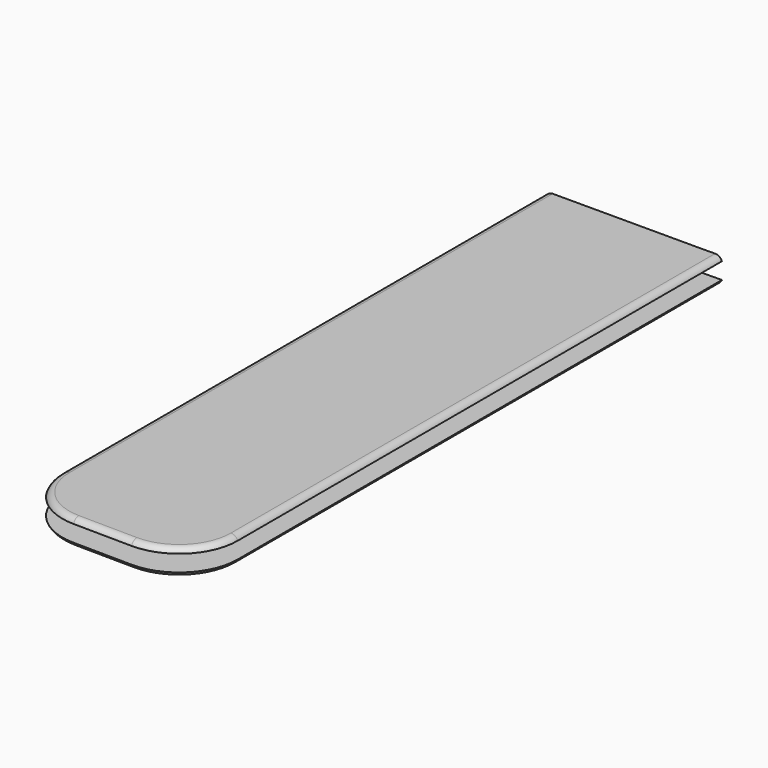
from build123d import *

# Parameters (mm, degrees)
F1_DEPTH        = 3.5
F2_DEPTH        = 2.25
F3_T1_DEPTH     = 169.9016407579
F3_T3_DEPTH     = 16.0006816658
F3_T5_DEPTH     = 169.6351240544
F3_T8_ANGLE     = 90.7094753215
F3_T10_ANGLE    = 89.290335423
F3_S1_T1_DEPTH  = 169.9016407579
F3_S1_T3_DEPTH  = 16.0006816658
F3_S1_T5_DEPTH  = 169.6351240544
F3_S1_T8_ANGLE  = 90.7094753215
F3_S1_T10_ANGLE = 89.290335423


# Not quite as in the source:
# - a fillet or chamfer that OpenCascade refuses, or shapes differently, is made with other operations: its cross-section is extruded or revolved along the edge and cut away or added


with BuildPart() as f1:
    # F0 (on Top) → F1 (new body, symmetric)
    with BuildSketch(Plane.XY):
        with BuildLine():
            Line((18, 42.4503772799), (-18, 42.4503772799))
            Line((-18, 42.4503772799), (-24.0000008941, 42.4503772799))
            Line((-24.0000008941, 42.4503772799), (-24.0000008941, -122.5496227201))
            ThreePointArc((-24.0000008941, -122.5496227201), (-19.3835574329, -133.7930496347), (-8.1981706793, -138.5483963291))
            Line((-8.1981706793, -138.5483963291), (7.8012836493, -138.7465754402))
            ThreePointArc((7.8012836493, -138.7465754402), (19.2428624423, -134.1313778333), (23.9994552225, -122.7478546813))
            Line((23.9994552225, -122.7478546813), (24.0000011197, 42.5186620212))
            Line((24.0000011197, 42.5186620212), (18, 42.4503772799))
        make_face()
    extrude(amount=F1_DEPTH, both=True)

    # F0 (on Top) → F2 (cut, symmetric)
    with BuildSketch(Plane.XY):
        with BuildLine():
            Line((18, 42.4503772799), (-18, 42.4503772799))
            Line((-18, 42.4503772799), (-24.0000008941, 42.4503772799))
            Line((-24.0000008941, 42.4503772799), (-24.0000008941, -122.5496227201))
            ThreePointArc((-24.0000008941, -122.5496227201), (-19.3835574329, -133.7930496347), (-8.1981706793, -138.5483963291))
            Line((-8.1981706793, -138.5483963291), (7.8012836493, -138.7465754402))
            ThreePointArc((7.8012836493, -138.7465754402), (19.2428624423, -134.1313778333), (23.9994552225, -122.7478546813))
            Line((23.9994552225, -122.7478546813), (24.0000011197, 42.5186620212))
            Line((24.0000011197, 42.5186620212), (18, 42.4503772799))
        make_face()
    extrude(amount=F2_DEPTH, both=True, mode=Mode.SUBTRACT)

    # F3: fillet of radius 2 on 1 edges, made by hand

    # F3_s2 → F3_t1 (cut)
    with BuildSketch(Plane(origin=(-0.0004054521, -122.7477754066, 0), x_dir=(0, 0, 1), z_dir=(3.3031e-06, 1, 0))):
        with BuildLine():
            ThreePointArc((-2.25, 23.9998606748), (-3.1583123952, 23.2638450417), (-3.5, 22.145811053))
            Line((-3.5, 22.145811053), (-3.5, 23.9998606748))
            Line((-3.5, 23.9998606748), (-2.25, 23.9998606748))
        make_face()
    extrude(amount=F3_T1_DEPTH, mode=Mode.SUBTRACT)

    # F3_s4 → F3_t3 (cut)
    with BuildSketch(Plane(origin=(-6.4810304011, 0.0802780406, 0), x_dir=(0, 0, 1), z_dir=(0.9999232947, -0.0123856668, 0))):
        with BuildLine():
            ThreePointArc((-3.5, 136.7852591194), (-3.1583123952, 137.9032931082), (-2.25, 138.6393087412))
            Line((-2.25, 138.6393087412), (-3.5, 138.6393087412))
            Line((-3.5, 138.6393087412), (-3.5, 136.7852591194))
        make_face()
    extrude(amount=F3_T3_DEPTH, mode=Mode.SUBTRACT)

    # F3_s6 → F3_t5 (cut)
    with BuildSketch(Plane.XZ.offset(-47.0855013343)):
        with BuildLine():
            ThreePointArc((-22.1459512723, -3.5), (-23.263985261, -3.1583123952), (-24.0000008941, -2.25))
            Line((-24.0000008941, -2.25), (-24.0000008941, -3.5))
            Line((-24.0000008941, -3.5), (-22.1459512723, -3.5))
        make_face()
    extrude(amount=F3_T5_DEPTH, mode=Mode.SUBTRACT)

    # F3_s7 → F3_t8 (revolve, cut)
    with BuildSketch(Plane(origin=(9.5184239274, -0.1179010705, 0), x_dir=(0, 0, 1), z_dir=(-0.9999232947, 0.0123856668, 0))):
        with BuildLine():
            ThreePointArc((-2.25, -138.6393087412), (-3.1583123952, -137.9032931082), (-3.5, -136.7852591194))
            Line((-3.5, -136.7852591194), (-3.5, -138.6393087412))
            Line((-3.5, -138.6393087412), (-2.25, -138.6393087412))
        make_face()
    revolve(axis=Axis((7.9994543285, -122.7478018312, -3.5), (0, 0, 1)), revolution_arc=F3_T8_ANGLE, mode=Mode.SUBTRACT)

    # F3_s9 → F3_t10 (revolve, cut)
    with BuildSketch(Plane.XZ.offset(122.5496227201)):
        with BuildLine():
            ThreePointArc((-22.1459512723, -3.5), (-23.263985261, -3.1583123952), (-24.0000008941, -2.25))
            Line((-24.0000008941, -2.25), (-24.0000008941, -3.5))
            Line((-24.0000008941, -3.5), (-22.1459512723, -3.5))
        make_face()
    revolve(axis=Axis((-8, -122.5496227201, -3.5), (0, 0, 1)), revolution_arc=F3_T10_ANGLE, mode=Mode.SUBTRACT)

    # F3#s1: fillet of radius 2 on 1 edges, made by hand

    # F3_s1_s2 → F3_s1_t1 (cut)
    with BuildSketch(Plane(origin=(-0.0004054521, -122.7477754066, 0), x_dir=(0, 0, 1), z_dir=(3.3031e-06, 1, 0))):
        with BuildLine():
            ThreePointArc((2.25, 23.9998606748), (3.1583123952, 23.2638450417), (3.5, 22.145811053))
            Line((3.5, 22.145811053), (3.5, 23.9998606748))
            Line((3.5, 23.9998606748), (2.25, 23.9998606748))
        make_face()
    extrude(amount=F3_S1_T1_DEPTH, mode=Mode.SUBTRACT)

    # F3_s1_s4 → F3_s1_t3 (cut)
    with BuildSketch(Plane(origin=(-6.4810304011, 0.0802780406, 0), x_dir=(0, 0, 1), z_dir=(0.9999232947, -0.0123856668, 0))):
        with BuildLine():
            ThreePointArc((3.5, 136.7852591194), (3.1583123952, 137.9032931082), (2.25, 138.6393087412))
            Line((2.25, 138.6393087412), (3.5, 138.6393087412))
            Line((3.5, 138.6393087412), (3.5, 136.7852591194))
        make_face()
    extrude(amount=F3_S1_T3_DEPTH, mode=Mode.SUBTRACT)

    # F3_s1_s6 → F3_s1_t5 (cut)
    with BuildSketch(Plane.XZ.offset(-47.0855013343)):
        with BuildLine():
            ThreePointArc((-22.1459512723, 3.5), (-23.263985261, 3.1583123952), (-24.0000008941, 2.25))
            Line((-24.0000008941, 2.25), (-24.0000008941, 3.5))
            Line((-24.0000008941, 3.5), (-22.1459512723, 3.5))
        make_face()
    extrude(amount=F3_S1_T5_DEPTH, mode=Mode.SUBTRACT)

    # F3_s1_s7 → F3_s1_t8 (revolve, cut)
    with BuildSketch(Plane(origin=(9.5184239274, -0.1179010705, 0), x_dir=(0, 0, 1), z_dir=(-0.9999232947, 0.0123856668, 0))):
        with BuildLine():
            ThreePointArc((2.25, -138.6393087412), (3.1583123952, -137.9032931082), (3.5, -136.7852591194))
            Line((3.5, -136.7852591194), (3.5, -138.6393087412))
            Line((3.5, -138.6393087412), (2.25, -138.6393087412))
        make_face()
    revolve(axis=Axis((7.9994543285, -122.7478018312, 3.5), (0, 0, 1)), revolution_arc=F3_S1_T8_ANGLE, mode=Mode.SUBTRACT)

    # F3_s1_s9 → F3_s1_t10 (revolve, cut)
    with BuildSketch(Plane.XZ.offset(122.5496227201)):
        with BuildLine():
            ThreePointArc((-22.1459512723, 3.5), (-23.263985261, 3.1583123952), (-24.0000008941, 2.25))
            Line((-24.0000008941, 2.25), (-24.0000008941, 3.5))
            Line((-24.0000008941, 3.5), (-22.1459512723, 3.5))
        make_face()
    revolve(axis=Axis((-8, -122.5496227201, 3.5), (0, 0, 1)), revolution_arc=F3_S1_T10_ANGLE, mode=Mode.SUBTRACT)


solid = f1.part
